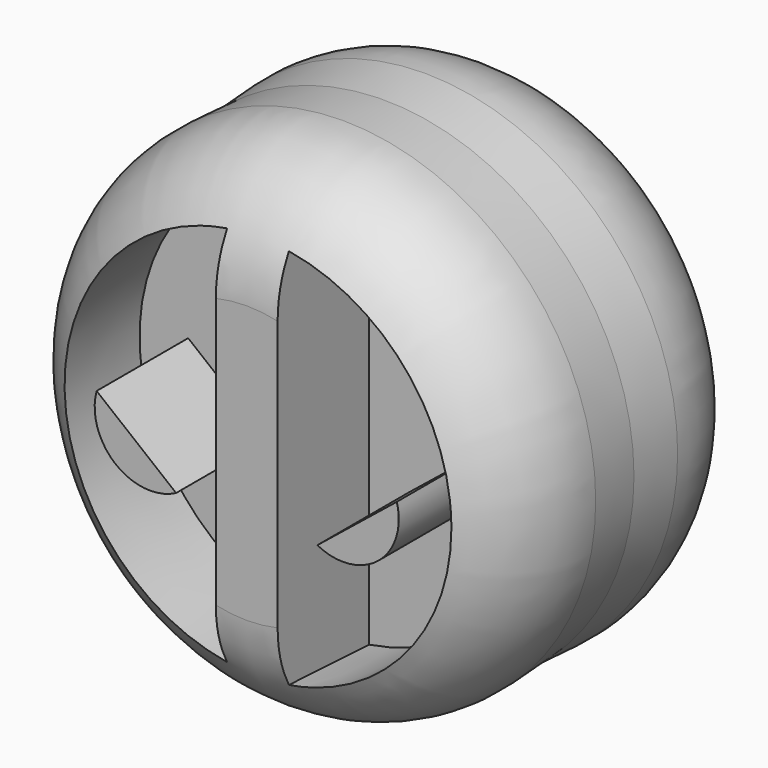
from build123d import *

# Parameters (mm, degrees)
F0_R         = 55.5262746105
F1_DEPTH     = 38.1
F1_TAPER     = -3
F2_DEPTH     = 38.1
F3_DEPTH     = 12.7
F4_DEPTH     = 38.1
F5_S5_R      = 12.3526687507
F5_T6_DEPTH  = 90
F5_S7_R      = 12.3526687507
F5_T8_DEPTH  = 90
F5_S13_R     = 12.3526687507
F5_T14_DEPTH = 90
F5_S15_R     = 12.3526687507
F5_T16_DEPTH = 90


# Not quite as in the source:
# - a fillet or chamfer that OpenCascade refuses, or shapes differently, is made with other operations: its cross-section is extruded or revolved along the edge and cut away or added
# - two fillets or chamfers of one size are made in one step


with BuildPart() as f1:
    # F0 (on Front) → F1 (new body, symmetric)
    with BuildSketch(Plane.XZ):
        Circle(F0_R)
        with BuildLine():
            ThreePointArc((6.861501839, 44.2620349836), (34.0113180152, 29.1451230097), (44.790712747, 0))
            ThreePointArc((44.790712747, 0), (34.0113180152, -29.1451230097), (6.861501839, -44.2620349836))
            Line((6.861501839, -44.2620349836), (6.861501839, -46.4376546443))
            Line((6.861501839, -46.4376546443), (-6.8615009077, -46.4376546443))
            Line((-6.8615009077, -46.4376546443), (-6.8615009077, -44.262035128))
            ThreePointArc((-6.8615009077, -44.262035128), (-44.790712747, 0), (-6.8615009077, 44.262035128))
            Line((-6.8615009077, 44.262035128), (-6.8615009077, 48.6431419849))
            Line((-6.8615009077, 48.6431419849), (6.861501839, 48.6431419849))
            Line((6.861501839, 48.6431419849), (6.861501839, 44.2620349836))
        make_face(mode=Mode.SUBTRACT)
        with BuildLine():
            ThreePointArc((-6.8615009077, 44.262035128), (4.712e-07, 44.790712747), (6.861501839, 44.2620349836))
            Line((6.861501839, 44.2620349836), (6.861501839, 48.6431419849))
            Line((6.861501839, 48.6431419849), (-6.8615009077, 48.6431419849))
            Line((-6.8615009077, 48.6431419849), (-6.8615009077, 44.262035128))
        make_face()
        with BuildLine():
            Line((6.861501839, -46.4376546443), (6.861501839, -44.2620349836))
            ThreePointArc((6.861501839, -44.2620349836), (4.712e-07, -44.790712747), (-6.8615009077, -44.262035128))
            Line((-6.8615009077, -44.262035128), (-6.8615009077, -46.4376546443))
            Line((-6.8615009077, -46.4376546443), (6.861501839, -46.4376546443))
        make_face()
    extrude(amount=F1_DEPTH, both=True, taper=F1_TAPER)

    # F0 (on Front) → F2 (join, symmetric)
    with BuildSketch(Plane.XZ):
        with BuildLine():
            Line((6.861501839, -44.2620349836), (6.861501839, 44.2620349836))
            ThreePointArc((6.861501839, 44.2620349836), (4.712e-07, 44.790712747), (-6.8615009077, 44.262035128))
            Line((-6.8615009077, 44.262035128), (-6.8615009077, -44.262035128))
            ThreePointArc((-6.8615009077, -44.262035128), (4.712e-07, -44.790712747), (6.861501839, -44.2620349836))
        make_face()
    extrude(amount=F2_DEPTH, both=True)

    # F0 (on Front) → F3 (join, symmetric)
    with BuildSketch(Plane.XZ):
        with BuildLine():
            Line((-6.8615009077, -44.262035128), (-6.8615009077, 44.262035128))
            ThreePointArc((-6.8615009077, 44.262035128), (-44.790712747, 0), (-6.8615009077, -44.262035128))
        make_face()
        with BuildLine():
            ThreePointArc((-15.6834311783, -10.942174576), (-29.1647493256, -9.6196886086), (-33.3272889256, 3.270934813))
            Line((-33.3272889256, 3.270934813), (-15.6834311783, -10.942174576))
        make_face(mode=Mode.SUBTRACT)
        with BuildLine():
            ThreePointArc((6.861501839, -44.2620349836), (34.0113180152, -29.1451230097), (44.790712747, 0))
            ThreePointArc((44.790712747, 0), (34.0113180152, 29.1451230097), (6.861501839, 44.2620349836))
            Line((6.861501839, 44.2620349836), (6.861501839, -44.2620349836))
        make_face()
        with BuildLine():
            Line((15.6834311783, -10.942174576), (33.3272889256, 3.270934813))
            ThreePointArc((33.3272889256, 3.270934813), (29.1647493256, -9.6196886086), (15.6834311783, -10.942174576))
        make_face(mode=Mode.SUBTRACT)
    extrude(amount=F3_DEPTH, both=True)

    # F0 (on Front) → F4 (join, symmetric)
    with BuildSketch(Plane.XZ):
        with BuildLine():
            Line((-15.6834311783, -10.942174576), (-33.3272889256, 3.270934813))
            ThreePointArc((-33.3272889256, 3.270934813), (-29.1647493256, -9.6196886086), (-15.6834311783, -10.942174576))
        make_face()
        with BuildLine():
            ThreePointArc((15.6834311783, -10.942174576), (29.1647493256, -9.6196886086), (33.3272889256, 3.270934813))
            Line((33.3272889256, 3.270934813), (15.6834311783, -10.942174576))
        make_face()
    extrude(amount=F4_DEPTH, both=True)

    # F5: fillet of radius 25.4 on 2 edges, made by hand


with BuildPart() as f5_tool2:
    # F5_s3 → F5_t4 (revolve)
    with BuildSketch(Plane.XY):
        with BuildLine():
            ThreePointArc((30.7569958191, 38.1), (49.1815048428, 30.1842062226), (56.1221860018, 11.3706667114))
            Line((56.1221860018, 11.3706667114), (57.5230110012, 38.1))
            Line((57.5230110012, 38.1), (30.7569958191, 38.1))
        make_face()
    revolve(axis=Axis((0, 38.1, 0), (0, -1, 0)))

    # F5_s5 → F5_t6 (cut, symmetric)
    with BuildSketch(Plane.XZ.offset(-16.4)):
        with Locations((-21.415554765, 0)):
            Circle(F5_S5_R)
    extrude(amount=F5_T6_DEPTH, both=True, mode=Mode.SUBTRACT)

    # F5_s7 → F5_t8 (cut, symmetric)
    with BuildSketch(Plane.XZ.offset(-16.4)):
        with Locations((21.415554765, 0)):
            Circle(F5_S7_R)
    extrude(amount=F5_T8_DEPTH, both=True, mode=Mode.SUBTRACT)


with BuildPart() as f1_1:
    add(f1.part)

    # F5_t1: cut F5_tool2
    add(f5_tool2.part, mode=Mode.SUBTRACT)


with BuildPart() as f5_tool10:
    # F5_s11 → F5_t12 (revolve)
    with BuildSketch(Plane.XY):
        with BuildLine():
            ThreePointArc((56.1221860018, -11.3706667114), (49.1815048428, -30.1842062226), (30.7569958191, -38.1))
            Line((30.7569958191, -38.1), (57.5230110012, -38.1))
            Line((57.5230110012, -38.1), (56.1221860018, -11.3706667114))
        make_face()
    revolve(axis=Axis((0, -38.1, 0), (0, 1, 0)))

    # F5_s13 → F5_t14 (cut, symmetric)
    with BuildSketch(Plane.XZ.offset(16.4)):
        with Locations((21.415554765, 0)):
            Circle(F5_S13_R)
    extrude(amount=F5_T14_DEPTH, both=True, mode=Mode.SUBTRACT)

    # F5_s15 → F5_t16 (cut, symmetric)
    with BuildSketch(Plane.XZ.offset(16.4)):
        with Locations((-21.415554765, 0)):
            Circle(F5_S15_R)
    extrude(amount=F5_T16_DEPTH, both=True, mode=Mode.SUBTRACT)


with BuildPart() as f1_2:
    add(f1_1.part)

    # F5_t9: cut F5_tool10
    add(f5_tool10.part, mode=Mode.SUBTRACT)


solid = f1_2.part
